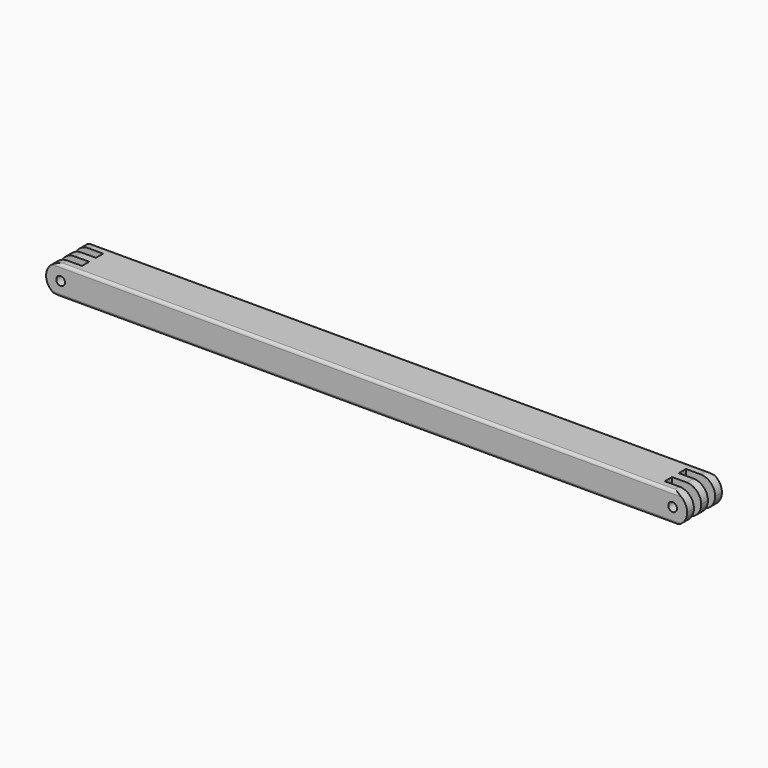
from build123d import *

# Parameters (mm, degrees)
F0_W        = 200
F0_H        = 10
F1_DEPTH    = 14.9
F2_W        = 10
F2_H        = 2.9
F3_DEPTH    = 10
F4_R        = 1.5
F5_DEPTH    = 14.9
F6_T1_DEPTH = 218.4999999506
F6_T3_DEPTH = 218.4999999928


# Not quite as in the source:
# - a fillet or chamfer that OpenCascade refuses, or shapes differently, is made with other operations: its cross-section is extruded or revolved along the edge and cut away or added


with BuildPart() as f1:
    # F0 (on Front) → F1 (new body)
    with BuildSketch(Plane.XZ):
        Rectangle(F0_W, F0_H)
    extrude(amount=F1_DEPTH)

    # F2 (on face) → F3 (join)
    with BuildSketch(Plane.XY.offset(5)):
        with Locations((-105, -13.45)):
            Rectangle(F2_W, F2_H)
        with Locations((-105, -7.45)):
            Rectangle(F2_W, F2_H)
        with Locations((-105, -1.45)):
            Rectangle(F2_W, F2_H)
        with Locations((105, -13.45)):
            Rectangle(F2_W, F2_H)
        with Locations((105, -7.45)):
            Rectangle(F2_W, F2_H)
        with Locations((105, -1.45)):
            Rectangle(F2_W, F2_H)
    extrude(amount=-F3_DEPTH)

    # F4 (on face) → F5 (cut)
    with BuildSketch(Plane(origin=(0, 0, 0), x_dir=(-1, 0, 0), z_dir=(0, 1, 0))):
        with BuildLine():
            ThreePointArc((-110, 0), (-108.5355339059, 3.5355339059), (-105, 5))
            Line((-105, 5), (-110, 5))
            Line((-110, 5), (-110, 0))
        make_face()
        with BuildLine():
            Line((-110, -5), (-105, -5))
            ThreePointArc((-105, -5), (-108.5355339059, -3.5355339059), (-110, 0))
            Line((-110, 0), (-110, -5))
        make_face()
        with Locations((-105, 0)):
            Circle(F4_R)
        with BuildLine():
            ThreePointArc((110, 0), (108.5355338885, -3.5355339234), (104.9999999506, -5))
            Line((104.9999999506, -5), (110, -5))
            Line((110, -5), (110, 0))
        make_face()
        with BuildLine():
            Line((110, 5), (104.9999999928, 5))
            ThreePointArc((104.9999999928, 5), (108.5355339034, 3.5355339085), (110, 0))
            Line((110, 0), (110, 5))
        make_face()
        with Locations((105, 0)):
            Circle(F4_R)
    extrude(amount=-F5_DEPTH, mode=Mode.SUBTRACT)

    # F6: fillet of radius 1 on 4 edges, made by hand

    # F6_s2 → F6_t1 (cut)
    with BuildSketch(Plane.YZ.offset(-109.2499999506)):
        with BuildLine():
            ThreePointArc((-1, -5), (-0.2928932188, -4.7071067812), (0, -4))
            Line((0, -4), (0, -5))
            Line((0, -5), (-1, -5))
        make_face()
        with BuildLine():
            ThreePointArc((-13.9, -5), (-14.6071067812, -4.7071067812), (-14.9, -4))
            Line((-14.9, -4), (-14.9, -5))
            Line((-14.9, -5), (-13.9, -5))
        make_face()
    extrude(amount=F6_T1_DEPTH, mode=Mode.SUBTRACT)

    # F6_s4 → F6_t3 (cut)
    with BuildSketch(Plane.YZ.offset(-109.2499999928)):
        with BuildLine():
            ThreePointArc((-1, 5), (-0.2928932188, 4.7071067812), (0, 4))
            Line((0, 4), (0, 5))
            Line((0, 5), (-1, 5))
        make_face()
        with BuildLine():
            ThreePointArc((-13.9, 5), (-14.6071067812, 4.7071067812), (-14.9, 4))
            Line((-14.9, 4), (-14.9, 5))
            Line((-14.9, 5), (-13.9, 5))
        make_face()
    extrude(amount=F6_T3_DEPTH, mode=Mode.SUBTRACT)


solid = f1.part
